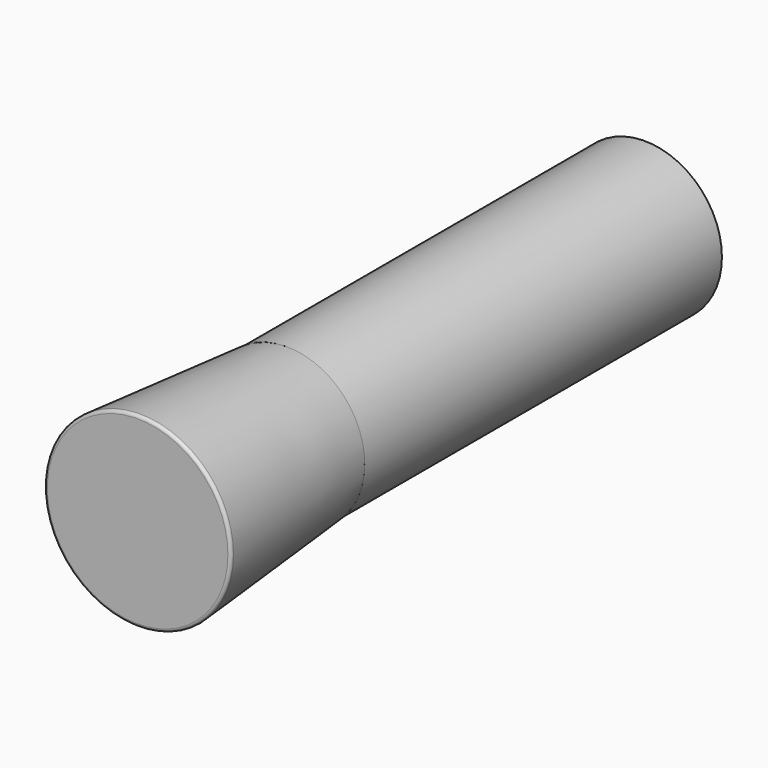
from build123d import *

# Parameters (mm, degrees)
F0_R     = 6.5786
F0_R_2   = 4.9911
F1_DEPTH = 14.0716
F3_START = 14.0716
F2_R     = 6.5786
F2_R_2   = 4.826
F3_DEPTH = 36.7284
F5_START = 38.1
F4_R     = 8.2296
F4_R_2   = 6.6421
F5_DEPTH = 12.7
F7_START = 50.8
F6_R     = 8.2296
F7_DEPTH = 3.175
F9_R     = 0.254


# Not quite as in the source:
# - a fillet or chamfer that OpenCascade refuses, or shapes differently, is made with other operations: its cross-section is extruded or revolved along the edge and cut away or added


with BuildPart() as f1:
    # F0 (on Front) → F1 (new body)
    with BuildSketch(Plane.XZ):
        Circle(F0_R)
        Circle(F0_R_2, mode=Mode.SUBTRACT)
    extrude(amount=F1_DEPTH)

    # F2 (on Front) → F3 (join)
    with BuildSketch(Plane.XZ.offset(F3_START)):
        Circle(F2_R)
        Circle(F2_R_2, mode=Mode.SUBTRACT)
    extrude(amount=F3_DEPTH)


with BuildPart() as f5:
    # F4 (on Front) → F5 (new body)
    with BuildSketch(Plane.XZ.offset(F5_START)):
        Circle(F4_R)
        Circle(F4_R_2, mode=Mode.SUBTRACT)
    extrude(amount=F5_DEPTH)

    # F6 (on Front) → F7 (join)
    with BuildSketch(Plane.XZ.offset(F7_START)):
        Circle(F6_R)
    extrude(amount=F7_DEPTH)

    # F8: chamfer of 19.05 x 1.5875 on 1 edges, made by hand

    # F8_s1 → F8_t2 (revolve, cut)
    with BuildSketch(Plane.XY):
        Polygon((8.2296, -57.15), (6.6421, -38.1), (8.2296, -38.1), align=None)
    revolve(axis=Axis((0, -38.1, 0), (0, -1, 0)), mode=Mode.SUBTRACT)

    # F9
    f9_edges = [f5.edges().sort_by_distance(p)[0] for p in [
        (-7.965017, -53.975, 0),
    ]]
    fillet(f9_edges, radius=F9_R)


solid = Compound([f1.part, f5.part])
